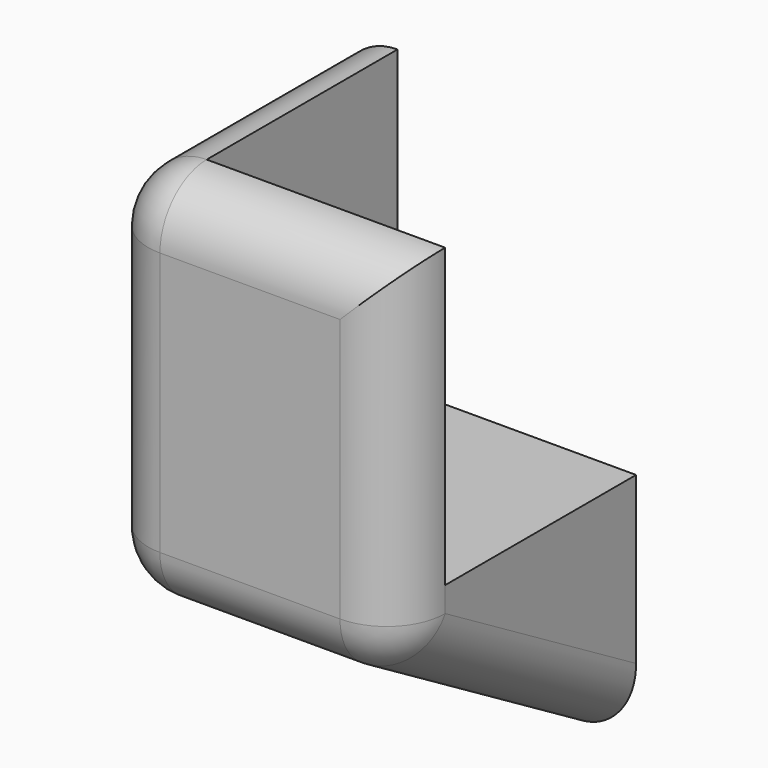
from build123d import *

# Parameters (mm, degrees)
F0_W     = 25.4
F0_H     = 25.4
F1_DEPTH = 5
F3_DEPTH = 25.4
F5_DEPTH = 25.4
F7_D     = 5
F9_D     = 10
F9_DEPTH = 20.4
F9_TIP   = 3.0043030951
F10_R    = 4.99999


# Not quite as in the source:
# - a fillet or chamfer is up to 0.001 mm smaller than in the source, because OpenCascade refuses the exact size


with BuildPart() as f1:
    # F0 (on Top) → F1 (new body)
    with BuildSketch(Plane.XY):
        with Locations((12.7, 12.7)):
            Rectangle(F0_W, F0_H)
    extrude(amount=F1_DEPTH)

    # F2 (on face) → F3 (join)
    with BuildSketch(Plane.XY.offset(5)):
        Polygon((5, 25.4), (0, 25.4), (0, 0), (25.4, 0), (25.4, 5), (5, 5), align=None)
    extrude(amount=F3_DEPTH)

    # F4 (on face) → F5 (join, through all)
    with BuildSketch(Plane.YZ.offset(25.4)):
        Polygon((25.4, -15), (25.4, 0), (0, 0), align=None)
    extrude(amount=-F5_DEPTH)

    # F7 (through all)
    with Locations(Plane.XZ):
        with Locations((12.7, -7.5)):
            Hole(F7_D / 2)

    # F9
    with Locations(Plane.XZ):
        with Locations((12.7, -7.5)):
            Hole(F9_D / 2, depth=F9_DEPTH)
            with Locations((0, 0, -(F9_DEPTH + F9_TIP / 2))):  # 118° drill point
                Cone(0, F9_D / 2, F9_TIP, mode=Mode.SUBTRACT)

    # F10 (radius 5 in the source; OpenCascade refuses exactly that, so slightly less here)
    f10_edges = [f1.edges().sort_by_distance(p)[0] for p in [
        (0, 0, 15.2),
        (0, 12.7, -7.5),
        (12.7, 0, 0),
        (25.4, 12.7, -7.5),
        (25.4, 0, 15.2),
        (12.7, 0, 30.4),
        (0, 12.7, 30.4),
    ]]
    fillet(f10_edges, radius=F10_R)


solid = f1.part
